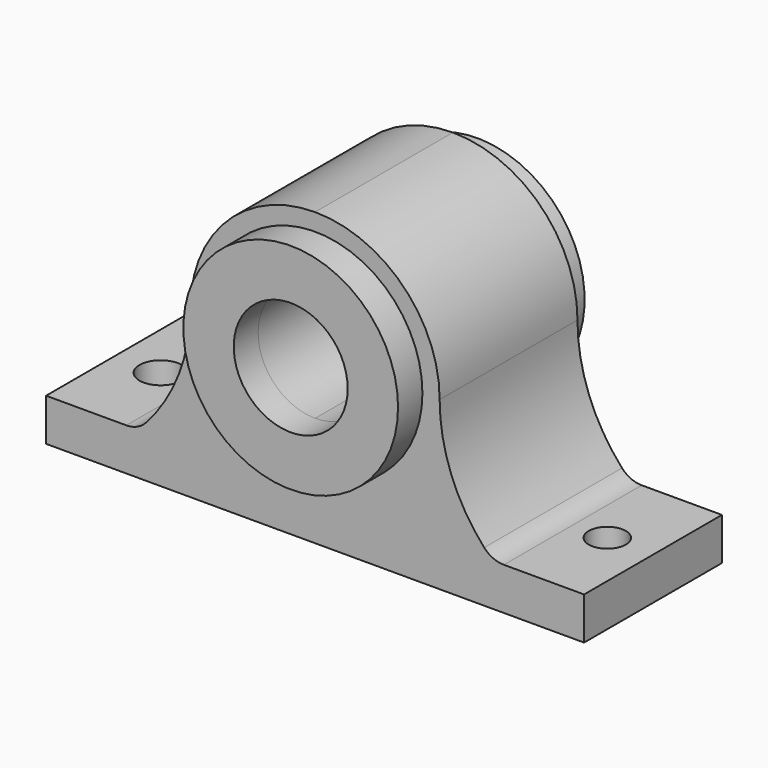
from build123d import *
from build123d import SkipClean  # not in build123d's __all__

# Parameters (mm, degrees)
F1_DEPTH = 65
F2_R     = 40.5
F2_R_2   = 21.5
F3_DEPTH = 11.5
F4_R     = 40.5
F4_R_2   = 21.5
F5_DEPTH = 11.5
F7_D     = 14
F9_R     = 10
F10_D    = 16


# Not quite as in the source:
# - after a boolean that leaves OpenCascade's solid faulty, fix() repairs it


with BuildPart() as f1:
    # F0 (on Front) → F1 (new body)
    with BuildSketch(Plane.XZ):
        with BuildLine():
            Line((0, 16), (0, 0))
            Line((0, 0), (101.5, 0))
            Line((101.5, 0), (101.5, 16))
            Line((101.5, 16), (67, 16))
            ThreePointArc((67, 16), (52.2079138911, 37.4608144218), (47, 63))
            ThreePointArc((47, 63), (33.2340187158, 96.2340187158), (0, 110))
            Line((0, 110), (0, 84.5))
            ThreePointArc((0, 84.5), (15.2027957955, 78.2027957955), (21.5, 63))
            ThreePointArc((21.5, 63), (15.2027957955, 47.7972042045), (0, 41.5))
            Line((0, 41.5), (0, 16))
        make_face()
        with BuildLine():
            Line((-101.5, 0), (0, 0))
            Line((0, 0), (0, 16))
            Line((0, 16), (0, 41.5))
            ThreePointArc((0, 41.5), (-21.5, 63), (0, 84.5))
            Line((0, 84.5), (0, 110))
            ThreePointArc((0, 110), (-33.2340187158, 96.2340187158), (-47, 63))
            ThreePointArc((-47, 63), (-52.2079138911, 37.4608144218), (-67, 16))
            Line((-67, 16), (-101.5, 16))
            Line((-101.5, 16), (-101.5, 0))
        make_face()
    extrude(amount=F1_DEPTH)

    # F2 (on face) → F3 (join)
    with BuildSketch(Plane.XZ.offset(65)):
        with Locations((0, 63)):
            Circle(F2_R)
        with Locations((0, 63)):
            Circle(F2_R_2, mode=Mode.SUBTRACT)
    extrude(amount=F3_DEPTH)

    # F4 (on face) → F5 (join)
    with BuildSketch(Plane(origin=(0, 0, 0), x_dir=(-1, 0, 0), z_dir=(0, 1, 0))):
        with Locations((0, 63)):
            Circle(F4_R)
        with Locations((0, 63)):
            Circle(F4_R_2, mode=Mode.SUBTRACT)
    with SkipClean():  # cleaning this boolean's faces spoils the solid; the shape is the same uncleaned
        extrude(amount=F5_DEPTH)

    # F7 (through all)
    with Locations(Plane.XY.offset(16)):
        with Locations((84.25, -32.5)):
            Hole(F7_D / 2)

    add(f1.part.fix(), mode=Mode.REPLACE)

    # F9
    f9_edges = [f1.edges().sort_by_distance(p)[0] for p in [
        (-67, -32.5, 16),
        (67, -32.5, 16),
    ]]
    fillet(f9_edges, radius=F9_R)

    # F10 (through all)
    with Locations(Plane.XY.offset(16)):
        with Locations((-84.25, -32.5)):
            Hole(F10_D / 2)


solid = f1.part
